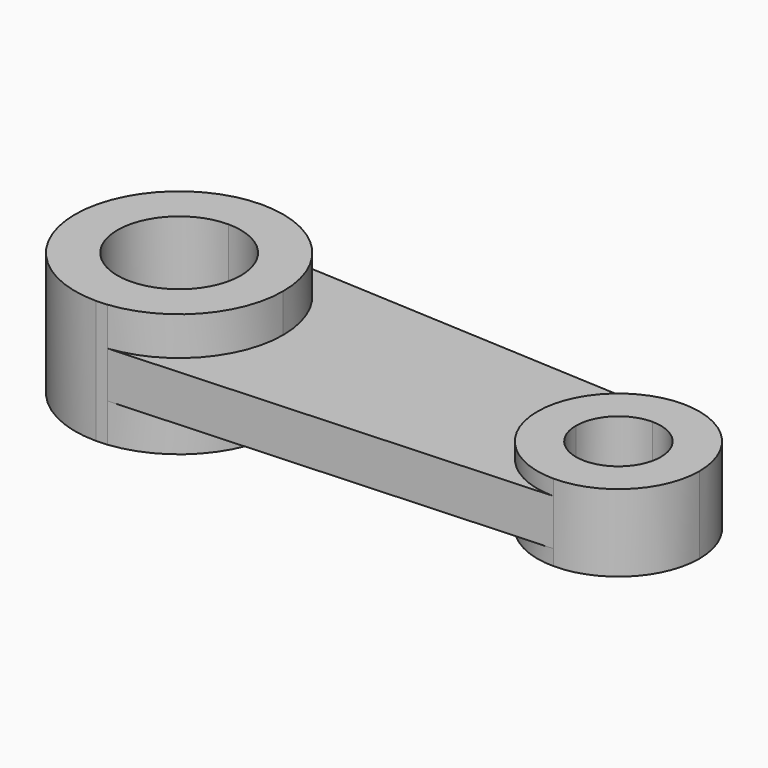
from build123d import *

# Parameters (mm, degrees)
F1_DEPTH      = 19.05
F2_DEPTH      = 15.875
F2_DEPTH_BACK = 34.925
F3_DEPTH      = 25.4
F3_DEPTH_BACK = 6.35


with BuildPart() as f1:
    # F0 (on Top) → F1 (new body)
    with BuildSketch(Plane.XY):
        with BuildLine():
            Line((4.499378, 42.625691), (0, 42.8625))
            Line((0, 42.8625), (0, 25.4))
            ThreePointArc((0, 25.4), (17.960512, 17.960512), (25.4, 0))
            Line((25.4, 0), (42.8625, 0))
            ThreePointArc((42.8625, 0), (31.859445, 28.673501), (4.499378, 42.625691))
        make_face()
        with BuildLine():
            Line((0, 25.4), (0, 42.8625))
            ThreePointArc((0, 42.8625), (-42.8625, 0), (0, -42.8625))
            Line((0, -42.8625), (0, -25.4))
            ThreePointArc((0, -25.4), (-25.4, 0), (0, 25.4))
        make_face()
        with BuildLine():
            Line((0, -25.4), (0, -42.8625))
            Line((0, -42.8625), (4.499378, -42.625691))
            ThreePointArc((4.499378, -42.625691), (31.859445, -28.673501), (42.8625, 0))
            Line((42.8625, 0), (25.4, 0))
            ThreePointArc((25.4, 0), (17.960512, -17.960512), (0, -25.4))
        make_face()
        with BuildLine():
            Line((180.975, 33.3375), (4.499378, 42.625691))
            ThreePointArc((4.499378, 42.625691), (31.859445, 28.673501), (42.8625, 0))
            Line((42.8625, 0), (147.6375, 0))
            ThreePointArc((147.6375, 0), (157.401828, 23.573172), (180.975, 33.3375))
        make_face()
        with BuildLine():
            ThreePointArc((42.8625, 0), (31.859445, -28.673501), (4.499378, -42.625691))
            Line((4.499378, -42.625691), (180.975, -33.3375))
            ThreePointArc((180.975, -33.3375), (157.401828, -23.573172), (147.6375, 0))
            Line((147.6375, 0), (42.8625, 0))
        make_face()
        with BuildLine():
            Line((180.975, 17.4625), (180.975, 33.3375))
            ThreePointArc((180.975, 33.3375), (157.401828, 23.573172), (147.6375, 0))
            Line((147.6375, 0), (163.5125, 0))
            ThreePointArc((163.5125, 0), (168.627148, 12.347852), (180.975, 17.4625))
        make_face()
        with BuildLine():
            ThreePointArc((147.6375, 0), (157.401828, -23.573172), (180.975, -33.3375))
            Line((180.975, -33.3375), (180.975, -17.4625))
            ThreePointArc((180.975, -17.4625), (168.627148, -12.347852), (163.5125, 0))
            Line((163.5125, 0), (147.6375, 0))
        make_face()
        with BuildLine():
            ThreePointArc((214.3125, 0), (204.548172, 23.573172), (180.975, 33.3375))
            Line((180.975, 33.3375), (180.975, 17.4625))
            ThreePointArc((180.975, 17.4625), (193.322852, 12.347852), (198.4375, 0))
            ThreePointArc((198.4375, 0), (193.322852, -12.347852), (180.975, -17.4625))
            Line((180.975, -17.4625), (180.975, -33.3375))
            ThreePointArc((180.975, -33.3375), (204.548172, -23.573172), (214.3125, 0))
        make_face()
    extrude(amount=F1_DEPTH)

    # F0 (on Top) → F2 (join, two sides)
    with BuildSketch(Plane.XY) as f2_sk:
        with BuildLine():
            Line((0, -25.4), (0, -42.8625))
            Line((0, -42.8625), (4.499378, -42.625691))
            ThreePointArc((4.499378, -42.625691), (31.859445, -28.673501), (42.8625, 0))
            Line((42.8625, 0), (25.4, 0))
            ThreePointArc((25.4, 0), (17.960512, -17.960512), (0, -25.4))
        make_face()
        with BuildLine():
            Line((0, 25.4), (0, 42.8625))
            ThreePointArc((0, 42.8625), (-42.8625, 0), (0, -42.8625))
            Line((0, -42.8625), (0, -25.4))
            ThreePointArc((0, -25.4), (-25.4, 0), (0, 25.4))
        make_face()
        with BuildLine():
            Line((4.499378, 42.625691), (0, 42.8625))
            Line((0, 42.8625), (0, 25.4))
            ThreePointArc((0, 25.4), (17.960512, 17.960512), (25.4, 0))
            Line((25.4, 0), (42.8625, 0))
            ThreePointArc((42.8625, 0), (31.859445, 28.673501), (4.499378, 42.625691))
        make_face()
    extrude(amount=-F2_DEPTH)
    extrude(f2_sk.sketch, amount=F2_DEPTH_BACK)

    # F0 (on Top) → F3 (join, two sides)
    with BuildSketch(Plane.XY) as f3_sk:
        with BuildLine():
            ThreePointArc((214.3125, 0), (204.548172, 23.573172), (180.975, 33.3375))
            Line((180.975, 33.3375), (180.975, 17.4625))
            ThreePointArc((180.975, 17.4625), (193.322852, 12.347852), (198.4375, 0))
            ThreePointArc((198.4375, 0), (193.322852, -12.347852), (180.975, -17.4625))
            Line((180.975, -17.4625), (180.975, -33.3375))
            ThreePointArc((180.975, -33.3375), (204.548172, -23.573172), (214.3125, 0))
        make_face()
        with BuildLine():
            ThreePointArc((147.6375, 0), (157.401828, -23.573172), (180.975, -33.3375))
            Line((180.975, -33.3375), (180.975, -17.4625))
            ThreePointArc((180.975, -17.4625), (168.627148, -12.347852), (163.5125, 0))
            Line((163.5125, 0), (147.6375, 0))
        make_face()
        with BuildLine():
            Line((180.975, 17.4625), (180.975, 33.3375))
            ThreePointArc((180.975, 33.3375), (157.401828, 23.573172), (147.6375, 0))
            Line((147.6375, 0), (163.5125, 0))
            ThreePointArc((163.5125, 0), (168.627148, 12.347852), (180.975, 17.4625))
        make_face()
    extrude(amount=F3_DEPTH)
    extrude(f3_sk.sketch, amount=-F3_DEPTH_BACK)


solid = f1.part
